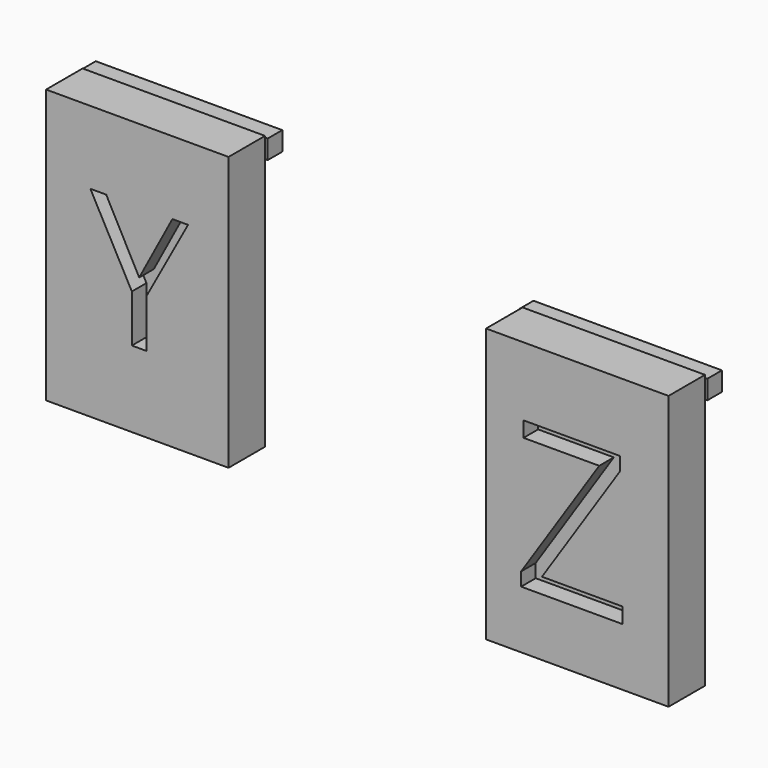
from build123d import *

# Parameters (mm, degrees)
F0_W           = 25.4
F0_H           = 38.1
F1_DEPTH       = 6.35
F2_R           = 3.81
F3_DEPTH       = 2.54
F5_TEXT_SIZE   = 24.2855968989
F5_TEXT_SIZE_2 = 28.7011602066
F6_DEPTH       = 25.4
F7_W           = 26.2284446508
F7_H           = 2.649336122
F8_DEPTH       = 2.54
F7_W_2         = 25.963511318
F7_H_2         = 2.6493389159


# Not quite as in the source:
# - Text() gives the source's letters only with a copy of the font that has no kerning and outlines rounded to 1/6400 em; it was checked with that copy


with BuildPart() as f1:
    # F0 (on Front) → F1 (new body)
    with BuildSketch(Plane.XZ):
        with Locations((-28.9658840819, 6.0590000916)):
            Rectangle(F0_W, F0_H)
    extrude(amount=F1_DEPTH)

    # F2 (on Front) → F3, piece 2 (join)
    with BuildSketch(Plane.XZ):
        with Locations((-34.0458840819, 14.9490000916)):
            Circle(F2_R)
        with Locations((-34.0458840819, -5.3709999084)):
            Circle(F2_R)
        with Locations((-23.8858840819, -5.3709999084)):
            Circle(F2_R)
        with Locations((-34.0458840819, 4.7890000916)):
            Circle(F2_R)
        with Locations((-23.8858840819, 14.9490000916)):
            Circle(F2_R)
    extrude(amount=-F3_DEPTH)


with BuildPart() as f1b:
    # F0 (on Front) → F1, piece 2 (new body)
    with BuildSketch(Plane.XZ):
        with Locations((32.2823398324, -3.3083746452)):
            Rectangle(F0_W, F0_H)
    extrude(amount=F1_DEPTH)

    # F2 (on Front) → F3 (join)
    with BuildSketch(Plane.XZ):
        with Locations((37.3623398324, 5.5816253548)):
            Circle(F2_R)
        with Locations((27.2023398324, -4.5783746452)):
            Circle(F2_R)
        with Locations((37.3623398324, -14.7383746452)):
            Circle(F2_R)
        with Locations((27.2023398324, -14.7383746452)):
            Circle(F2_R)
    extrude(amount=-F3_DEPTH)


with BuildPart() as f6_tool:
    # F5 (on offset) → F6 (new body)
    with BuildSketch(Plane.XZ.offset(3.81)):
        with Locations((-35.5011243373, -2.3844011594)):
            Text('Y', F5_TEXT_SIZE, font='Open Sans', text_align=(TextAlign.LEFT, TextAlign.BOTTOM))
        with Locations((23.3141668141, -14.3064232543)):
            Text('Z', F5_TEXT_SIZE_2, font='Open Sans', text_align=(TextAlign.LEFT, TextAlign.BOTTOM))
    extrude(amount=F6_DEPTH)


with BuildPart() as f1_1:
    add(f1.part)

    # F6: cut by f6_tool
    add(f6_tool.part, mode=Mode.SUBTRACT)

    # F7 (on Front) → F8, piece 2 (join)
    with BuildSketch(Plane.XZ):
        with Locations((-28.8777817041, 23.5791066661)):
            Rectangle(F7_W_2, F7_H_2)
    extrude(amount=-F8_DEPTH)


with BuildPart() as f1b_1:
    add(f1b.part)

    # F6: cut by f6_tool
    add(f6_tool.part, mode=Mode.SUBTRACT)

    # F7 (on Front) → F8 (join)
    with BuildSketch(Plane.XZ):
        with Locations((32.189453952, 14.0414903872)):
            Rectangle(F7_W, F7_H)
    extrude(amount=-F8_DEPTH)


solid = Compound([f1_1.part, f1b_1.part])
